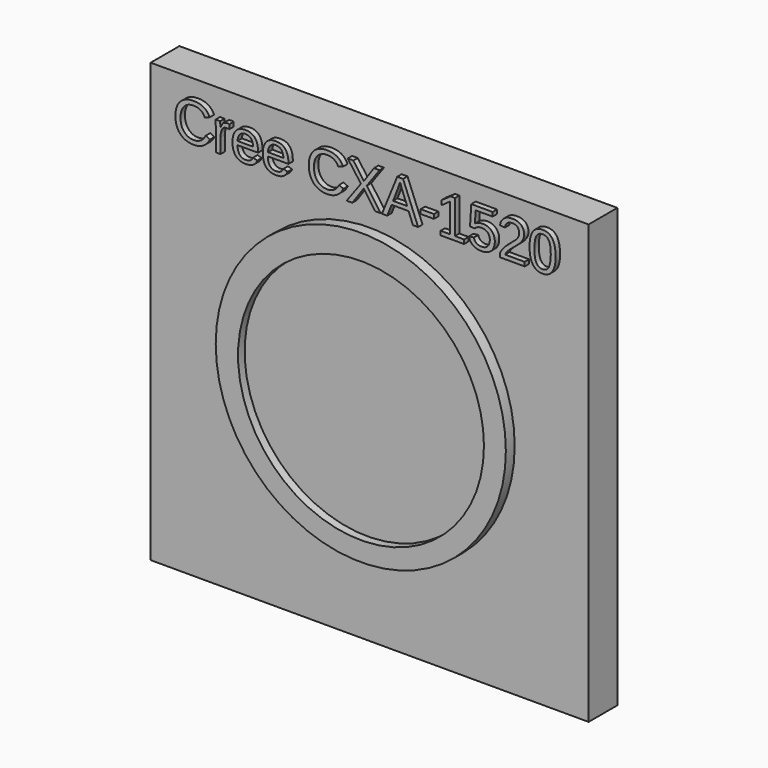
from build123d import *

# Parameters (mm, degrees)
F1_R         = 4.45
F2_DEPTH     = 1.4
F1_R_2       = 5.25
F3_DEPTH     = 1.7
F0_W         = 15.85
F0_H         = 15.85
F4_DEPTH     = 1.3
F5_TEXT_SIZE = 1.9748732643
F6_DEPTH     = 0.2


# Not quite as in the source:
# - Text() gives the source's letters only with a copy of the font that has no kerning and outlines rounded to 1/6400 em; it was checked with that copy


with BuildPart() as f2:
    # F1 (on face) → F2 (new body)
    with BuildSketch(Plane.XZ):
        with Locations((0.0071981112, -0.098979041)):
            Circle(F1_R)
    extrude(amount=F2_DEPTH)

    # F1 (on face) → F3 (join)
    with BuildSketch(Plane.XZ):
        Circle(F1_R_2)
        with Locations((0.0071981112, -0.098979041)):
            Circle(F1_R, mode=Mode.SUBTRACT)
    extrude(amount=F3_DEPTH)

    # F0 (on Front) → F4 (join)
    with BuildSketch(Plane.XZ):
        Rectangle(F0_W, F0_H)
    extrude(amount=F4_DEPTH)

    # F5 (on face) → F6 (join)
    with BuildSketch(Plane.XZ.offset(1.3)):
        with Locations((-6.9710501373, 5.9677093038)):
            Text('Cree CXA-1520', F5_TEXT_SIZE, font='Arimo', text_align=(TextAlign.LEFT, TextAlign.BOTTOM))
    extrude(amount=F6_DEPTH)


solid = f2.part
